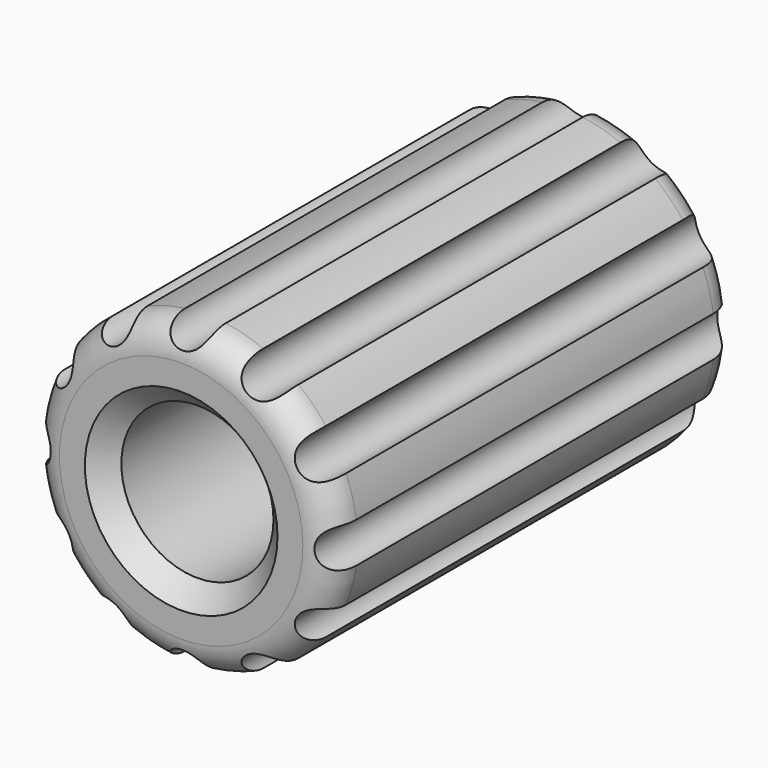
from build123d import *

# Parameters (mm, degrees)
F0_R     = 7.5
F0_R_2   = 3.75
F1_DEPTH = 25
F2_DEPTH = 2
F4_R     = 1.5
F5_R     = 1.5
F6_DEPTH = 25
F7_SIZE  = 1


with BuildPart() as f1:
    # F0 (on Front) → F1 (new body)
    with BuildSketch(Plane.XZ):
        Circle(F0_R)
        Circle(F0_R_2, mode=Mode.SUBTRACT)
    extrude(amount=F1_DEPTH)

    # F0 (on Front) → F2 (join)
    with BuildSketch(Plane.XZ):
        Circle(F0_R_2)
    extrude(amount=F2_DEPTH)

    # F4
    f4_edges = [f1.edges().sort_by_distance(p)[0] for p in [
        (-7.5, 0, 0),
    ]]
    fillet(f4_edges, radius=F4_R)

    # F5
    f5_edges = [f1.edges().sort_by_distance(p)[0] for p in [
        (-7.5, -25, 0),
    ]]
    fillet(f5_edges, radius=F5_R)

    # F3 (on face) → F6 (cut)
    with BuildSketch(Plane.XZ):
        with BuildLine():
            ThreePointArc((0.9977753031, 7.4333333333), (0, 7.5), (-0.9977753031, 7.4333333333))
            ThreePointArc((-0.9977753031, 7.4333333333), (0, 6.5), (0.9977753031, 7.4333333333))
        make_face()
        with BuildLine():
            ThreePointArc((-4.5807654265, 5.9385678499), (-3.75, 6.4951905284), (-2.8525679069, 6.936343153))
            ThreePointArc((-2.8525679069, 6.936343153), (-4.25, 7.3612159322), (-4.5807654265, 5.9385678499))
        make_face()
        with BuildLine():
            ThreePointArc((-2.75, 6.4951905284), (-2.7759794424, 6.721650135), (-2.8525679069, 6.936343153))
            ThreePointArc((-2.8525679069, 6.936343153), (-3.75, 6.4951905284), (-4.5807654265, 5.9385678499))
            ThreePointArc((-4.5807654265, 5.9385678499), (-3.4591094935, 5.5384341784), (-2.75, 6.4951905284))
        make_face()
        with BuildLine():
            ThreePointArc((4.5807654265, 5.9385678499), (3.75, 6.4951905284), (2.8525679069, 6.936343153))
            ThreePointArc((2.8525679069, 6.936343153), (3.25, 5.6291651246), (4.5807654265, 5.9385678499))
        make_face()
        with BuildLine():
            ThreePointArc((-6.936343153, 2.8525679069), (-6.4951905284, 3.75), (-5.9385678499, 4.5807654265))
            ThreePointArc((-5.9385678499, 4.5807654265), (-7.3612159322, 4.25), (-6.936343153, 2.8525679069))
        make_face()
        with BuildLine():
            ThreePointArc((-5.4951905284, 3.75), (-5.6129709756, 4.2208382533), (-5.9385678499, 4.5807654265))
            ThreePointArc((-5.9385678499, 4.5807654265), (-6.4951905284, 3.75), (-6.936343153, 2.8525679069))
            ThreePointArc((-6.936343153, 2.8525679069), (-5.9665851106, 2.9011323352), (-5.4951905284, 3.75))
        make_face()
        with BuildLine():
            ThreePointArc((6.936343153, 2.8525679069), (6.4951905284, 3.75), (5.9385678499, 4.5807654265))
            ThreePointArc((5.9385678499, 4.5807654265), (5.6291651246, 3.25), (6.936343153, 2.8525679069))
        make_face()
        with BuildLine():
            ThreePointArc((-7.4333333333, -0.9977753031), (-7.5, 0), (-7.4333333333, 0.9977753031))
            ThreePointArc((-7.4333333333, 0.9977753031), (-8.5, 0), (-7.4333333333, -0.9977753031))
        make_face()
        with BuildLine():
            ThreePointArc((-6.5, 0), (-6.7697032567, 0.6831300511), (-7.4333333333, 0.9977753031))
            ThreePointArc((-7.4333333333, 0.9977753031), (-7.5, 0), (-7.4333333333, -0.9977753031))
            ThreePointArc((-7.4333333333, -0.9977753031), (-6.7697032567, -0.6831300511), (-6.5, 0))
        make_face()
        with BuildLine():
            ThreePointArc((7.5, 0), (7.4833147735, 0.5), (7.4333333333, 0.9977753031))
            ThreePointArc((7.4333333333, 0.9977753031), (6.5, 0), (7.4333333333, -0.9977753031))
            ThreePointArc((7.4333333333, -0.9977753031), (7.4833147735, -0.5), (7.5, 0))
        make_face()
        with BuildLine():
            ThreePointArc((8.5, 0), (8.1831300511, 0.7302967433), (7.4333333333, 0.9977753031))
            ThreePointArc((7.4333333333, 0.9977753031), (7.4833147735, 0.5), (7.5, 0))
            ThreePointArc((7.5, 0), (7.4833147735, -0.5), (7.4333333333, -0.9977753031))
            ThreePointArc((7.4333333333, -0.9977753031), (8.1831300511, -0.7302967433), (8.5, 0))
        make_face()
        with BuildLine():
            ThreePointArc((-5.4951905284, -3.75), (-5.9665851106, -2.9011323352), (-6.936343153, -2.8525679069))
            ThreePointArc((-6.936343153, -2.8525679069), (-6.4951905284, -3.75), (-5.9385678499, -4.5807654265))
            ThreePointArc((-5.9385678499, -4.5807654265), (-5.6129709756, -4.2208382533), (-5.4951905284, -3.75))
        make_face()
        with BuildLine():
            ThreePointArc((5.9385678499, -4.5807654265), (6.4951905284, -3.75), (6.936343153, -2.8525679069))
            ThreePointArc((6.936343153, -2.8525679069), (5.6291651246, -3.25), (5.9385678499, -4.5807654265))
        make_face()
        with BuildLine():
            ThreePointArc((-2.75, -6.4951905284), (-3.4591094935, -5.5384341784), (-4.5807654265, -5.9385678499))
            ThreePointArc((-4.5807654265, -5.9385678499), (-3.75, -6.4951905284), (-2.8525679069, -6.936343153))
            ThreePointArc((-2.8525679069, -6.936343153), (-2.7759794424, -6.721650135), (-2.75, -6.4951905284))
        make_face()
        with BuildLine():
            ThreePointArc((2.8525679069, -6.936343153), (3.75, -6.4951905284), (4.5807654265, -5.9385678499))
            ThreePointArc((4.5807654265, -5.9385678499), (3.25, -5.6291651246), (2.8525679069, -6.936343153))
        make_face()
        with BuildLine():
            ThreePointArc((0.9977753031, -7.4333333333), (0, -6.5), (-0.9977753031, -7.4333333333))
            ThreePointArc((-0.9977753031, -7.4333333333), (0, -7.5), (0.9977753031, -7.4333333333))
        make_face()
    extrude(amount=F6_DEPTH, mode=Mode.SUBTRACT)

    # F7
    f7_edges = [f1.edges().sort_by_distance(p)[0] for p in [
        (-3.75, -25, 0),
    ]]
    chamfer(f7_edges, length=F7_SIZE)


solid = f1.part
